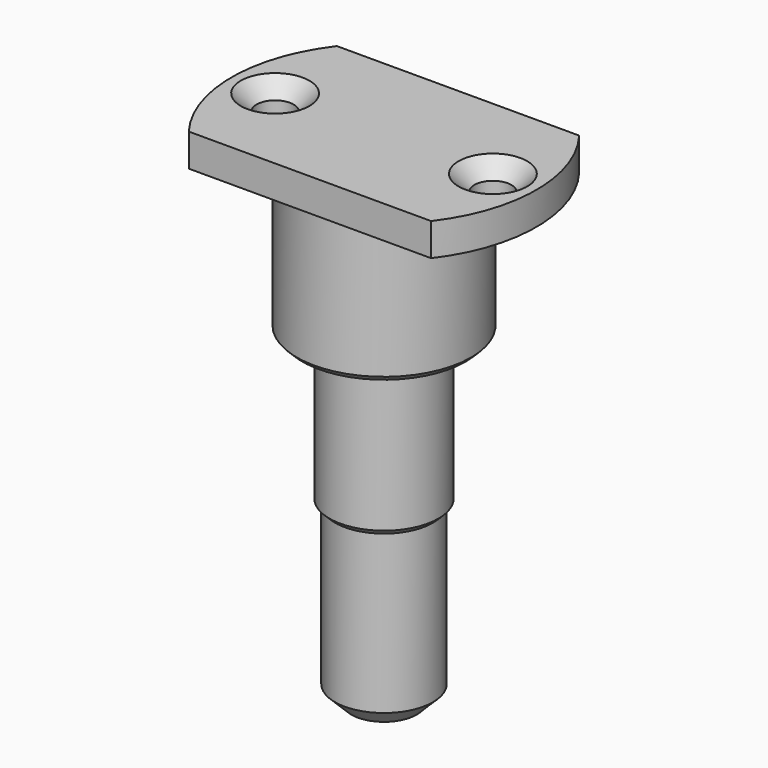
from build123d import *

# Parameters (mm, degrees)
F2_R            = 4.5
F3_DEPTH        = 46
F1_R            = 5
F4_DEPTH        = 30
F0_R            = 8
F5_DEPTH        = 16
F6_SIZE2        = 1.5
F6_SIZE         = 1.5
F7_SIZE2        = 0.49999
F7_SIZE         = 0.49999
F8_SIZE2        = 0.5
F8_SIZE         = 0.5
F10_DEPTH       = 3
F12_D           = 3.4
F12_CSINK_D     = 6.3
F12_CSINK_ANGLE = 90
F13_D           = 3.4
F13_CSINK_D     = 6.3
F13_CSINK_ANGLE = 90
F15_R           = 0.5


# Not quite as in the source:
# - a fillet or chamfer is up to 0.001 mm smaller than in the source, because OpenCascade refuses the exact size
# - a feature of the source that left no trace in its solid (it failed there, or was rolled back) is left out


with BuildPart() as f3:
    # F2 (on Top) → F3 (new body)
    with BuildSketch(Plane.XY):
        Circle(F2_R)
    extrude(amount=-F3_DEPTH)

    # F1 (on Top) → F4 (join)
    with BuildSketch(Plane.XY):
        Circle(F1_R)
    extrude(amount=-F4_DEPTH)

    # F0 (on Top) → F5 (join)
    with BuildSketch(Plane.XY):
        Circle(F0_R)
    extrude(amount=-F5_DEPTH)

    # F6
    f6_edges = [f3.edges().sort_by_distance(p)[0] for p in [
        (-4.5, 0, -46),
    ]]
    chamfer(f6_edges, length=F6_SIZE, length2=F6_SIZE2)

    # F7 (size 0.5 and 0.5 in the source; OpenCascade refuses exactly that, so slightly less here)
    f7_edges = [f3.edges().sort_by_distance(p)[0] for p in [
        (-5, 0, -30),
    ]]
    chamfer(f7_edges, length=F7_SIZE, length2=F7_SIZE2)

    # F8
    f8_edges = [f3.edges().sort_by_distance(p)[0] for p in [
        (-8, 0, -16),
    ]]
    chamfer(f8_edges, length=F8_SIZE, length2=F8_SIZE2)

    # F9 (on Top) → F10 (join)
    with BuildSketch(Plane.XY):
        with BuildLine():
            Line((11.1242977306, 8.5), (-11.1242977306, 8.5))
            ThreePointArc((-11.1242977306, 8.5), (-14, 0), (-11.1242977306, -8.5))
            Line((-11.1242977306, -8.5), (11.1242977306, -8.5))
            ThreePointArc((11.1242977306, -8.5), (14, 0), (11.1242977306, 8.5))
        make_face()
    extrude(amount=-F10_DEPTH)

    # F12 (through all)
    with Locations(Plane.XY):
        with Locations((-10, 0)):
            CounterSinkHole(F12_D / 2, F12_CSINK_D / 2, counter_sink_angle=F12_CSINK_ANGLE)

    # F13 (through all)
    with Locations(Plane.XY):
        with Locations((10, 0)):
            CounterSinkHole(F13_D / 2, F13_CSINK_D / 2, counter_sink_angle=F13_CSINK_ANGLE)

    # F15
    f15_edges = [f3.edges().sort_by_distance(p)[0] for p in [
        (-5, 0, -16),
    ]]
    fillet(f15_edges, radius=F15_R)


solid = f3.part
